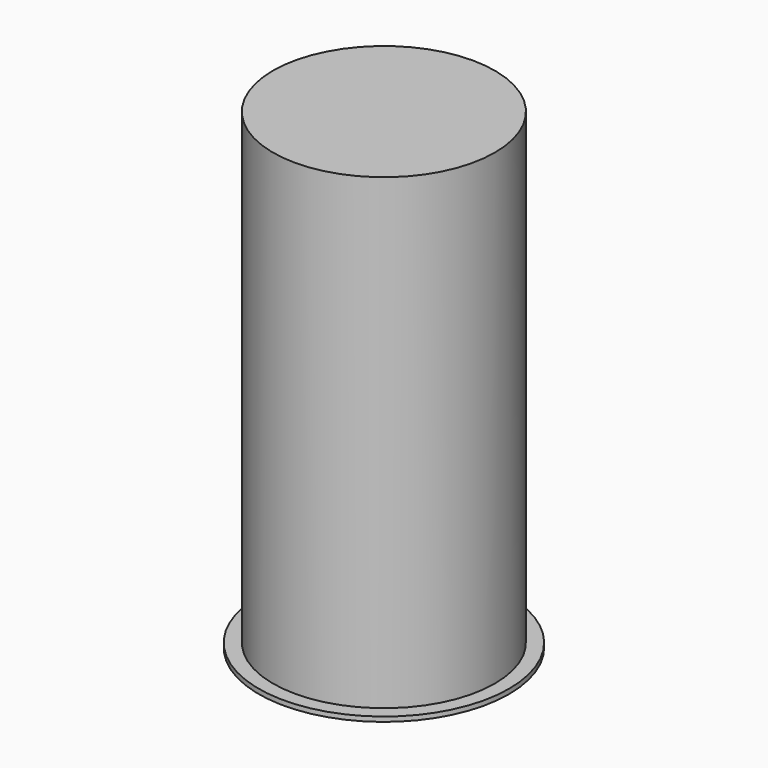
from build123d import *

# Parameters (mm, degrees)
F0_R     = 53
F0_R_2   = 47
F1_DEPTH = 2
F2_DEPTH = 200
F3_T     = 2


# Not quite as in the source:
# - a shell that OpenCascade refuses in one call is made with other operations: the cavity is built on its own and cut out


with BuildPart() as f1:
    # F0 (on Top) → F1 (new body)
    with BuildSketch(Plane.XY):
        Circle(F0_R)
        Circle(F0_R_2, mode=Mode.SUBTRACT)
    extrude(amount=F1_DEPTH)

    # F0 (on Top) → F2 (join)
    with BuildSketch(Plane.XY):
        Circle(F0_R_2)
    extrude(amount=F2_DEPTH)

    # F3: shell of thickness 2, made by hand


with BuildPart() as f3_core1:
    # F3_t2: copy of F1
    add(f1.part)

    # the walls: a layer under each face that stays
    f3_faces = [f3_core1.faces().sort_by_distance(p)[0] for p in [
        (-53, 0, 1),
        (-35.3333333333, -35.3333333333, 2),
        (-47, 0, 101),
        (0, 0, 200),
    ]]
    thicken(f3_faces, amount=-F3_T, mode=Mode.SUBTRACT)

    # F3_s3 → F3_t4 (revolve, cut)
    with BuildSketch(Plane.XZ):
        Polygon((47.02, 2.02), (47, 0), (45, 0), (45, 2), align=None)
    revolve(axis=Axis((0, 0, 2), (0, 0, 1)), mode=Mode.SUBTRACT)


with BuildPart() as f1_1:
    add(f1.part)

    # what is left inside the walls is the cavity
    f3_cavity = [f3_core1.part.solids().sort_by_distance(p)[0] for p in [
        (-44.98, 0, 132.666667),
    ]]
    add(f3_cavity, mode=Mode.SUBTRACT)


solid = f1_1.part
